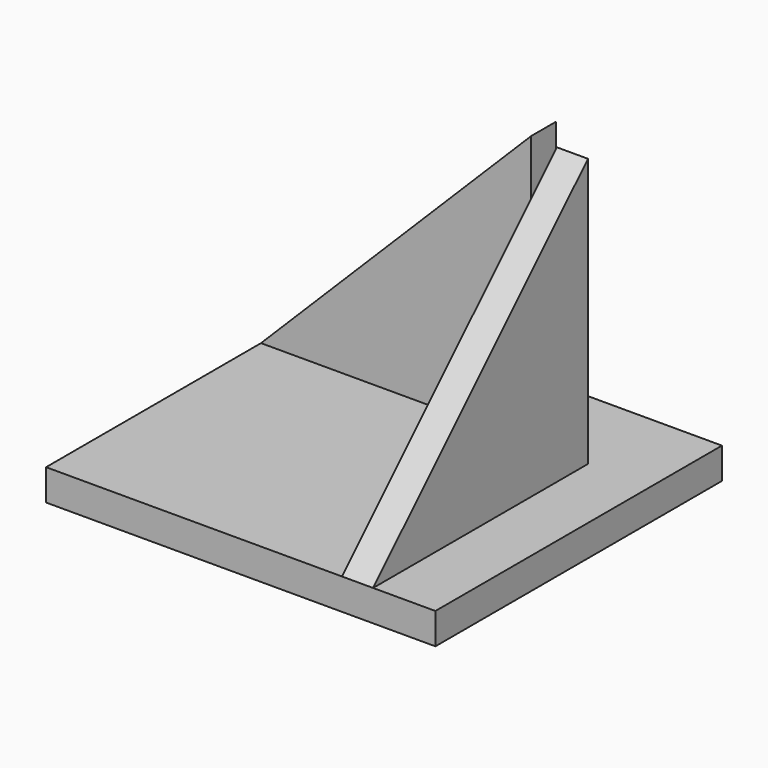
from build123d import *

# Parameters (mm, degrees)
F0_W     = 250
F0_H     = 230
F1_DEPTH = 20
F3_DEPTH = 57.5
F4_DEPTH = 37.5
F6_DEPTH = 60
F7_DEPTH = 40


with BuildPart() as f1:
    # F0 (on Top) → F1 (new body)
    with BuildSketch(Plane.XY):
        Rectangle(F0_W, F0_H)
    extrude(amount=F1_DEPTH)



with BuildPart() as f3:
    # F2 (on face) → F3 (new body)
    with BuildSketch(Plane(origin=(0, 115, 0), x_dir=(-1, 0, 0), z_dir=(0, 1, 0))):
        Polygon((-48.5, 20), (125, 20), (-48.5, 193.5), align=None)
    extrude(amount=-F3_DEPTH)

    # F4 (cut): a face of the model
    f4_faces = [f3.faces().sort_by_distance(p)[0] for p in [
        (-9.3333333333, 115, 77.8333333333),
    ]]
    extrude(f4_faces, amount=-F4_DEPTH, mode=Mode.SUBTRACT)


with BuildPart() as f1_1:
    add(f1.part)

    add(f3.part)  # F6 merges F3
    # F5 (on face) → F6 (join)
    with BuildSketch(Plane.YZ.offset(125)):
        Polygon((57.5, 192.5), (-115, 20), (57.5, 20), align=None)
    extrude(amount=-F6_DEPTH)

    # F5 (on face) → F7 (cut)
    with BuildSketch(Plane.YZ.offset(125)):
        Polygon((57.5, 192.5), (-115, 20), (57.5, 20), align=None)
    extrude(amount=-F7_DEPTH, mode=Mode.SUBTRACT)


solid = f1_1.part
